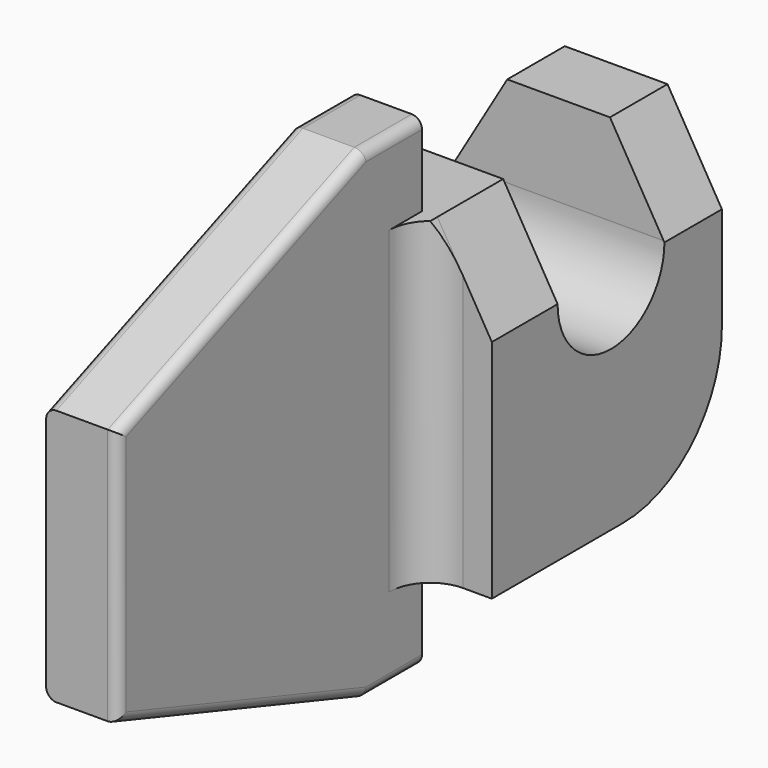
from build123d import *

# Parameters (mm, degrees)
F0_W          = 5.15
F0_H          = 11
F1_DEPTH      = 14
F3_DEPTH      = 5.151
F3_DEPTH_BACK = 5.151
F5_DEPTH      = 1.75
F6_R          = 6
F7_T4_DEPTH   = 15.5
F7_T9_DEPTH   = 15.5
F8_R          = 0.5


# Not quite as in the source:
# - a fillet or chamfer that OpenCascade refuses, or shapes differently, is made with other operations: its cross-section is extruded or revolved along the edge and cut away or added


with BuildPart() as f1:
    # F0 (on Front) → F1 (new body)
    with BuildSketch(Plane.XZ):
        with Locations((2.575, 0)):
            Rectangle(F0_W, F0_H)
        Polygon((0, 5.5), (5.15, 5.5), (2.5, 10), (0, 10), align=None)
        with Locations((-2.575, 0)):
            Rectangle(F0_W, F0_H)
        Polygon((-5.15, 5.5), (0, 5.5), (0, 10), (-2.5, 10), align=None)
    extrude(amount=-F1_DEPTH)

    # F2 (on Right) → F3 (cut, two sides)
    with BuildSketch(Plane.YZ) as f3_sk:
        with BuildLine():
            Line((4.0006404915, 10), (4.0006404915, 5.5))
            ThreePointArc((4.0006404915, 5.5), (7.2844648336, 2.2498275803), (10.5006404915, 5.5669554351))
            Line((10.5006404915, 5.5669554351), (10.5, 10))
            Line((10.5, 10), (4.0006404915, 10))
        make_face()
    extrude(amount=F3_DEPTH, mode=Mode.SUBTRACT)
    extrude(f3_sk.sketch, amount=-F3_DEPTH_BACK, mode=Mode.SUBTRACT)

    # F4 (on Right) → F5 (join, symmetric)
    with BuildSketch(Plane.YZ):
        Polygon((0, -9.5), (0, 0), (0, 14), (-3.5, 14), (-18.5, 8), (-18.5, -4.5), (-3.5, -9.5), align=None)
    extrude(amount=F5_DEPTH, both=True)

    # F6
    f6_edges = [f1.edges().sort_by_distance(p)[0] for p in [
        (0, 14, -5.5),
    ]]
    fillet(f6_edges, radius=F6_R)

    # F7: fillet of radius 2 on 2 edges, made by hand


with BuildPart() as f7_tool2:
    # F7_s3 → F7_t4 (new body)
    with BuildSketch(Plane.XY.offset(10)):
        with BuildLine():
            ThreePointArc((3.75, 0), (2.3357864376, -0.5857864376), (1.75, -2))
            Line((1.75, -2), (1.75, 0))
            Line((1.75, 0), (3.75, 0))
        make_face()
    extrude(amount=-F7_T4_DEPTH)

    split(bisect_by=Plane(origin=(6.2288019067, 0, 3.6680722339), x_dir=(0, 1, 0), z_dir=(-0.8616879874, 0, -0.5074384814)), keep=Keep.TOP)


with BuildPart() as f1_1:
    add(f1.part)

    # F7_t1: union F7_tool2
    add(f7_tool2.part)


with BuildPart() as f7_tool7:
    # F7_s8 → F7_t9 (new body)
    with BuildSketch(Plane.XY.offset(-5.5)):
        with BuildLine():
            ThreePointArc((-3.75, 0), (-2.3357864376, -0.5857864376), (-1.75, -2))
            Line((-1.75, -2), (-1.75, 0))
            Line((-1.75, 0), (-3.75, 0))
        make_face()
    extrude(amount=F7_T9_DEPTH)

    split(bisect_by=Plane(origin=(-6.2288019067, 0, 3.6680722339), x_dir=(0, 1, 0), z_dir=(0.8616879874, 0, -0.5074384814)), keep=Keep.TOP)


with BuildPart() as f1_2:
    add(f1_1.part)

    # F7_t6: union F7_tool7
    add(f7_tool7.part)

    # F8
    f8_edges = [f1_2.edges().sort_by_distance(p)[0] for p in [
        (1.75, -11, 11),
        (1.75, -1.75, 14),
        (1.75, -18.5, 1.75),
        (1.75, -11, -7),
        (1.75, -1.75, -9.5),
        (-1.75, -11, 11),
        (-1.75, -1.75, 14),
        (-1.75, -11, -7),
    ]]
    fillet(f8_edges, radius=F8_R)


solid = f1_2.part
